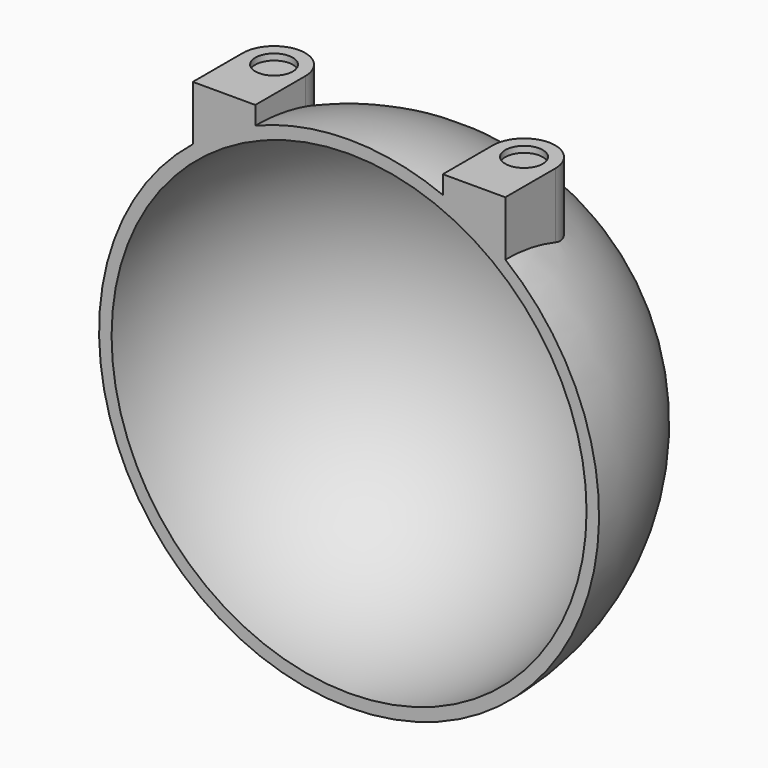
from build123d import *

# Parameters (mm, degrees)
F1_ANGLE = 180
F3_DEPTH = 40
F6_R     = 3
F7_DEPTH = 1


# Not quite as in the source:
# - a pattern or mirror of a feature is missing from the dataset's text; its kind, count and spacing are read off the source's solid


with BuildPart() as f1:
    # F0 (on Front) → F1 (revolve)
    with BuildSketch(Plane.XZ):
        with BuildLine():
            Line((0, 0), (0, -40))
            ThreePointArc((0, -40), (40, 0), (0, 40))
            Line((0, 40), (0, 0))
        make_face()
    revolve(axis=Axis((0, 0, 20), (0, 0, 1)), revolution_arc=F1_ANGLE)

    # F2 (on Top) → F3 (join)
    with BuildSketch(Plane.XY):
        with BuildLine():
            Line((-25, 0), (-15, 0))
            Line((-15, 0), (-15, 10))
            ThreePointArc((-15, 10), (-20, 15), (-25, 10))
            Line((-25, 10), (-25, 0))
        make_face()
        with BuildLine():
            Line((15, 10), (15, 0))
            Line((15, 0), (25, 0))
            Line((25, 0), (25, 10))
            ThreePointArc((25, 10), (20, 15), (15, 10))
        make_face()
    extrude(amount=F3_DEPTH)

    # F4 (on face) → F5 (revolve, cut)
    with BuildSketch(Plane.XZ):
        with BuildLine():
            Line((0, 38), (0, -38))
            ThreePointArc((0, -38), (38, 0), (0, 38))
        make_face()
    revolve(axis=Axis((0, 0, 0), (0, 0, 1)), mode=Mode.SUBTRACT)

    # F6 (on face) → F7 (cut)
    with BuildSketch(Plane.XY.offset(40)):
        with Locations((20, 10)):
            Circle(F6_R)
    f7 = extrude(amount=-F7_DEPTH, mode=Mode.SUBTRACT)

    # F7_copies: F7 across plane
    add(f7.mirror(Plane(origin=(0, 0, 0), x_dir=(0, 0, -1), z_dir=(-1, 0, 0))), mode=Mode.SUBTRACT)


solid = f1.part
